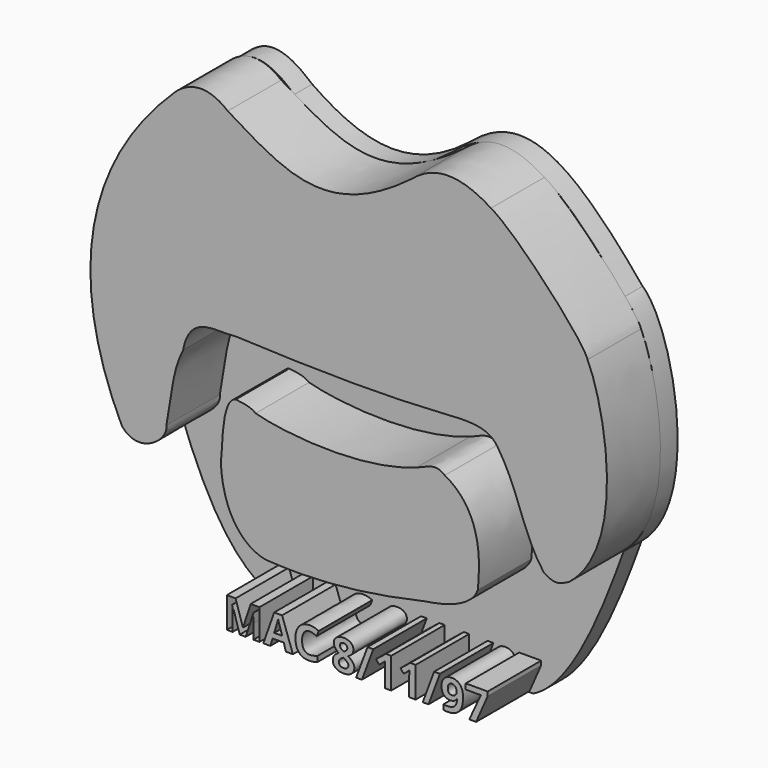
from build123d import *

# Parameters (mm, degrees)
F1_DEPTH     = 5
F3_DEPTH     = 15
F4_TEXT_SIZE = 9.6105716288
F5_DEPTH     = 15


# Not quite as in the source:
# - Text() gives the source's letters only with a copy of the font that has no kerning and outlines rounded to 1/6400 em; it was checked with that copy


with BuildPart() as f1:
    # F0 (on Front) → F1 (new body)
    with BuildSketch(Plane.XZ):
        with BuildLine():
            add(Edge.make_bspline(
                [(-41.6872054338, 36.0075384378), (-64.716629684, 10.3902416304), (-55.0722666085, -16.8026033789), (-49.6375635266, -27.9276203364)],
                knots=[0, 0, 0, 0, 64.4275773353, 64.4275773353, 64.4275773353, 64.4275773353], degree=3))
            add(Edge.make_bspline(
                [(-49.6375635266, -27.9276203364), (-45.7305163145, -38.0570068955), (-39.16176036, -57.7898845077), (-26.7170835286, -61.8416406214)],
                knots=[0, 0, 0, 0, 40.9329839522, 40.9329839522, 40.9329839522, 40.9329839522], degree=3))
            Line((-26.7170835286, -61.8416406214), (31.0142356902, -61.8416406214))
            add(Edge.make_bspline(
                [(31.0142356902, -61.8416406214), (40.2753880868, -57.2592994819), (47.3301000893, -37.9894599319), (51.2781143188, -27.1456036717)],
                knots=[0, 0, 0, 0, 40.1800915516, 40.1800915516, 40.1800915516, 40.1800915516], degree=3))
            add(Edge.make_bspline(
                [(51.2781143188, -27.1456036717), (65.1499032974, -15.8291431144), (58.4573745728, 17.390139401), (51.5214800835, 23.2308916748)],
                knots=[0, 0, 0, 0, 50.3770831856, 50.3770831856, 50.3770831856, 50.3770831856], degree=3))
            add(Edge.make_bspline(
                [(12.65351365, 39.0495993197), (24.064123513, 48.991007946), (34.1209024191, 44.5253066719), (51.5214800835, 23.2308916748)],
                knots=[0, 0, 0, 0, 41.9636786546, 41.9636786546, 41.9636786546, 41.9636786546], degree=3))
            add(Edge.make_bspline(
                [(12.65351365, 39.0495993197), (0, 29.1560341814), (-10.2931587026, 30.531834811), (-22.5830730051, 39.0495993197)],
                knots=[0, 0, 0, 0, 35.2365866551, 35.2365866551, 35.2365866551, 35.2365866551], degree=3))
            add(Edge.make_bspline(
                [(-22.5830730051, 39.0495993197), (-33.2911238074, 48.4191402793), (-36.8513688445, 40.3241030872), (-41.6872054338, 36.0075384378)],
                knots=[0, 0, 0, 0, 19.344818693, 19.344818693, 19.344818693, 19.344818693], degree=3))
        make_face()
    extrude(amount=F1_DEPTH)

    # F4 (on face) → F5 (join)
    with BuildSketch(Plane.XZ.offset(5)):
        with Locations((-26.6063413024, -61.6045603491)):
            Text('MAC 8/11/97', F4_TEXT_SIZE, font='Open Sans', font_style=FontStyle.BOLD, text_align=(TextAlign.LEFT, TextAlign.BOTTOM))
    extrude(amount=F5_DEPTH)


with BuildPart() as f3:
    # F2 (on face) → F3 (new body)
    with BuildSketch(Plane.XZ.offset(5)):
        with BuildLine():
            add(Edge.make_bspline(
                [(-49.270298332, -29.029045254), (-59.2343918979, -8.651625365), (-61.444927007, 17.6889989525), (-37.2475162148, 40.9142784774)],
                knots=[0, 0, 0, 0, 70.9691188084, 70.9691188084, 70.9691188084, 70.9691188084], degree=3))
            add(Edge.make_bspline(
                [(-39.3062010407, -25.6587583572), (-38.7731231749, -28.5127907991), (-45.2955216169, -33.7760131806), (-49.270298332, -29.029045254)],
                knots=[0, 0, 0, 0, 10.5186533642, 10.5186533642, 10.5186533642, 10.5186533642], degree=3))
            add(Edge.make_bspline(
                [(-35.5203337967, -9.4827832654), (-38.0890928209, -14.4890965894), (-38.0890928209, -19.6792818606), (-39.3062010407, -25.6587583572)],
                knots=[0, 0, 0, 0, 16.6130960678, 16.6130960678, 16.6130960678, 16.6130960678], degree=3))
            add(Edge.make_bspline(
                [(-23.4746243805, -3.0160555616), (-28.118474409, -3.5623910371), (-33.9915789664, -1.3770494843), (-35.5203337967, -9.4827832654)],
                knots=[0, 0, 0, 0, 13.6717841753, 13.6717841753, 13.6717841753, 13.6717841753], degree=3))
            add(Edge.make_bspline(
                [(24.1931024939, -3.0160555616), (7.9396562651, -4.108726047), (-7.9040685669, -3.6989748478), (-23.4746243805, -3.0160555616)],
                knots=[0, 0, 0, 0, 47.6677268744, 47.6677268744, 47.6677268744, 47.6677268744], degree=3))
            add(Edge.make_bspline(
                [(36.4068882602, -8.0920449224), (34.4326781171, -4.8130863112), (34.0271703899, -2.1965522319), (24.1931024939, -3.0160555616)],
                knots=[0, 0, 0, 0, 13.2265729022, 13.2265729022, 13.2265729022, 13.2265729022], degree=3))
            add(Edge.make_bspline(
                [(45.3976504505, -27.2193960845), (41.0332418978, -21.4767549187), (39.9995669723, -14.5281571895), (36.4068882602, -8.0920449224)],
                knots=[0, 0, 0, 0, 21.1350270225, 21.1350270225, 21.1350270225, 21.1350270225], degree=3))
            add(Edge.make_bspline(
                [(50.9680137038, -27.2193960845), (48.716455698, -28.3679254353), (47.8669852018, -28.7124831229), (45.3976504505, -27.2193960845)],
                knots=[0, 0, 0, 0, 5.5703632534, 5.5703632534, 5.5703632534, 5.5703632534], degree=3))
            add(Edge.make_bspline(
                [(55.1683716476, 18.0507916957), (58.7884373963, 10.8012976125), (64.5368546247, -16.5542867035), (50.9680137038, -27.2193960845)],
                knots=[0, 0, 0, 0, 45.4646336015, 45.4646336015, 45.4646336015, 45.4646336015], degree=3))
            add(Edge.make_bspline(
                [(33.4856845438, 40.9142784774), (38.3013114333, 38.5393276811), (54.1368946433, 21.7123199254), (55.1683716476, 18.0507916957)],
                knots=[0, 0, 0, 0, 31.5099658498, 31.5099658498, 31.5099658498, 31.5099658498], degree=3))
            add(Edge.make_bspline(
                [(15.7099347562, 40.9142784774), (18.8537277281, 43.6244420707), (24.4908705354, 46.764601022), (33.4856845438, 40.9142784774)],
                knots=[0, 0, 0, 0, 17.7757497877, 17.7757497877, 17.7757497877, 17.7757497877], degree=3))
            add(Edge.make_bspline(
                [(-25.5394149572, 40.9142784774), (-12.8010157496, 33.2174040377), (-3.4780441783, 26.3877846301), (15.7099347562, 40.9142784774)],
                knots=[0, 0, 0, 0, 41.2493497133, 41.2493497133, 41.2493497133, 41.2493497133], degree=3))
            add(Edge.make_bspline(
                [(-37.2475162148, 40.9142784774), (-35.2411940694, 42.757190764), (-30.9049282223, 45.3589484096), (-25.5394149572, 40.9142784774)],
                knots=[0, 0, 0, 0, 11.7081012577, 11.7081012577, 11.7081012577, 11.7081012577], degree=3))
        make_face()
    extrude(amount=F3_DEPTH)


with BuildPart() as f3b:
    # F2 (on face) → F3, piece 2 (new body)
    with BuildSketch(Plane.XZ.offset(5)):
        with BuildLine():
            add(Edge.make_bspline(
                [(23.1500323862, -15.2048217133), (32.5762666762, -20.2724356204), (30.7685676962, -32.6707400382), (30.5515099317, -35.4201458395)],
                knots=[0, 0, 0, 0, 21.5276844873, 21.5276844873, 21.5276844873, 21.5276844873], degree=3))
            add(Edge.make_bspline(
                [(23.1500323862, -15.2048217133), (20.9984816611, -13.3344838396), (18.8912320882, -15.0168742985), (16.8202947825, -15.7071873546)],
                knots=[0, 0, 0, 0, 6.3496416725, 6.3496416725, 6.3496416725, 6.3496416725], degree=3))
            add(Edge.make_bspline(
                [(16.8202947825, -15.7071873546), (4.4656926766, -20.2827481553), (-12.520189397, -18.6201203614), (-19.2883815616, -16.7508088052)],
                knots=[0, 0, 0, 0, 36.1237546922, 36.1237546922, 36.1237546922, 36.1237546922], degree=3))
            add(Edge.make_bspline(
                [(-19.2883815616, -16.7508088052), (-20.5775629729, -15.7194659114), (-22.2269458075, -15.6793591256), (-23.7360522151, -15.4616301879)],
                knots=[0, 0, 0, 0, 4.6307403025, 4.6307403025, 4.6307403025, 4.6307403025], degree=3))
            add(Edge.make_bspline(
                [(-27.0881783217, -29.029045254), (-26.6342740506, -26.3962540776), (-27.0966589451, -16.2204774097), (-23.7360522151, -15.4616301879)],
                knots=[0, 0, 0, 0, 13.9753891184, 13.9753891184, 13.9753891184, 13.9753891184], degree=3))
            add(Edge.make_bspline(
                [(-16.9351715595, -44.9322611094), (-21.1055353284, -44.2833527923), (-26.5258681029, -39.8386791348), (-27.0881783217, -29.029045254)],
                knots=[0, 0, 0, 0, 18.8678515167, 18.8678515167, 18.8678515167, 18.8678515167], degree=3))
            add(Edge.make_bspline(
                [(18.8584756106, -41.4905622602), (5.6709083728, -44.5001646876), (-5.4949773476, -45.6926375628), (-16.9351715595, -44.9322611094)],
                knots=[0, 0, 0, 0, 35.9587328573, 35.9587328573, 35.9587328573, 35.9587328573], degree=3))
            add(Edge.make_bspline(
                [(30.5515099317, -35.4201458395), (29.1044544429, -39.6166071296), (22.1487190574, -41.03115201), (18.8584756106, -41.4905622602)],
                knots=[0, 0, 0, 0, 13.1748626996, 13.1748626996, 13.1748626996, 13.1748626996], degree=3))
        make_face()
    extrude(amount=F3_DEPTH)


solid = Compound([f1.part, f3.part, f3b.part])
